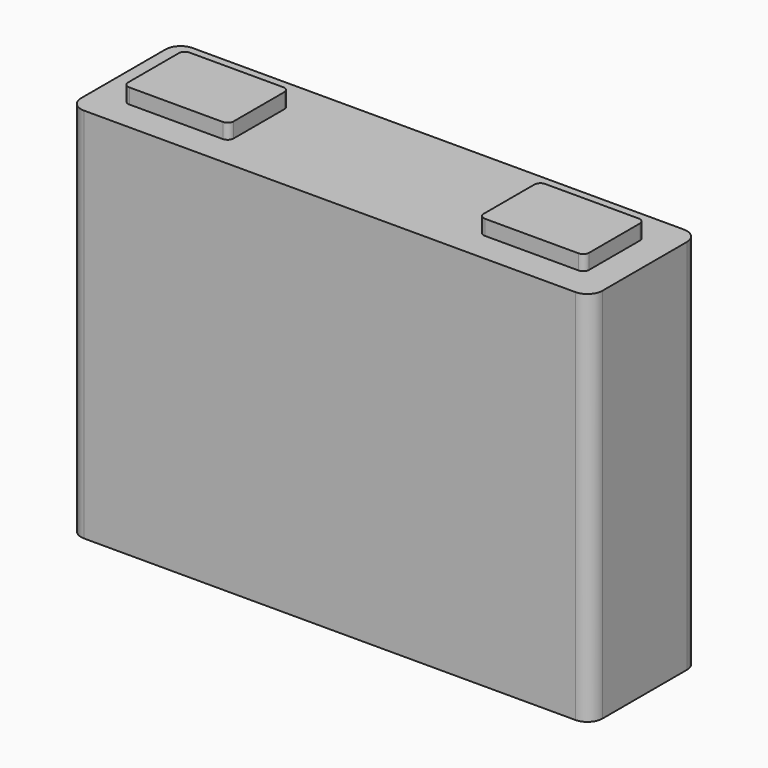
from build123d import *

# Parameters (mm, degrees)
F0_W     = 173
F0_H     = 125
F1_DEPTH = 45
F2_R     = 5
F3_R     = 5
F5_DEPTH = 5


# Not quite as in the source:
# - a pattern or mirror of a feature is missing from the dataset's text; its kind, count and spacing are read off the source's solid


with BuildPart() as f1:
    # F0 (on Front) → F1 (new body)
    with BuildSketch(Plane.XZ):
        with Locations((-86.5, 62.5)):
            Rectangle(F0_W, F0_H)
    extrude(amount=-F1_DEPTH)

    # F2
    f2_edges = [f1.edges().sort_by_distance(p)[0] for p in [
        (0, 0, 62.5),
    ]]
    fillet(f2_edges, radius=F2_R)

    # F3
    f3_edges = [f1.edges().sort_by_distance(p)[0] for p in [
        (0, 45, 62.5),
        (-173, 45, 62.5),
        (-173, 0, 62.5),
    ]]
    fillet(f3_edges, radius=F3_R)

    # F4 (on face) → F5 (join)
    with BuildSketch(Plane.XY.offset(125)):
        with BuildLine():
            Line((-130, 35), (-161, 35))
            ThreePointArc((-161, 35), (-162.4142135624, 34.4142135624), (-163, 33))
            Line((-163, 33), (-163, 12))
            ThreePointArc((-163, 12), (-162.4142135624, 10.5857864376), (-161, 10))
            Line((-161, 10), (-130, 10))
            ThreePointArc((-130, 10), (-128.5857864376, 10.5857864376), (-128, 12))
            Line((-128, 12), (-128, 33))
            ThreePointArc((-128, 33), (-128.5857864376, 34.4142135624), (-130, 35))
        make_face()
    f5 = extrude(amount=F5_DEPTH)

    # F5_copies: F5 across plane
    add(f5.mirror(Plane(origin=(-86.5, 0, 0), x_dir=(0, 0, 1), z_dir=(1, 0, 0))))


solid = f1.part
